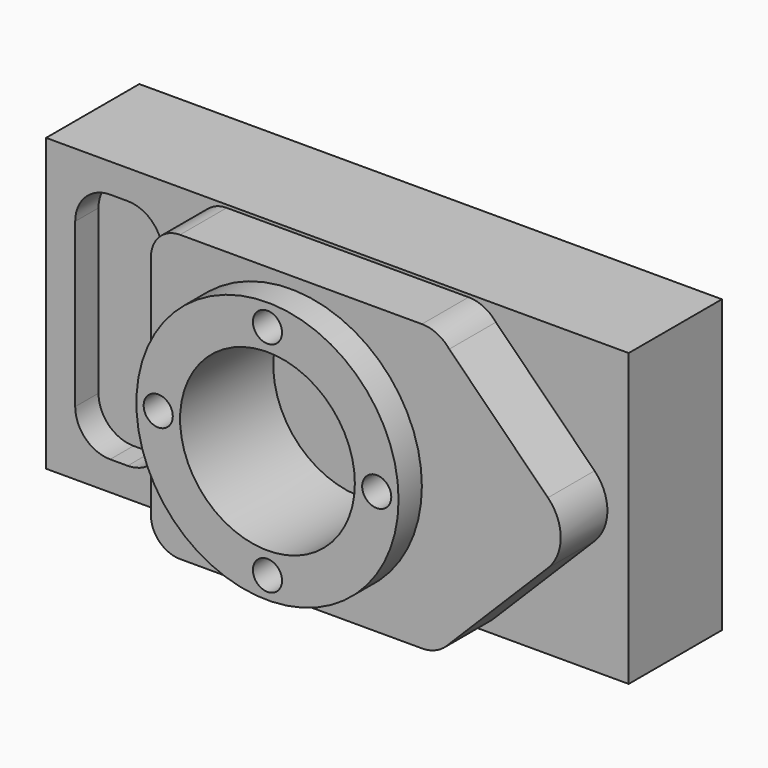
from build123d import *

# Parameters (mm, degrees)
F0_W     = 200
F0_H     = 100
F1_DEPTH = 40
F2_R     = 30
F3_DEPTH = 10
F4_R     = 30
F5_DEPTH = 20
F6_R     = 45
F6_R_2   = 30
F7_DEPTH = 10
F8_R     = 5
F9_DEPTH = 25


with BuildPart() as f1:
    # F0 (on Front) → F1 (new body)
    with BuildSketch(Plane.XZ):
        with Locations((-100, 50)):
            Rectangle(F0_W, F0_H)
    extrude(amount=F1_DEPTH)

    # F2 (on face) → F3 (cut)
    with BuildSketch(Plane.XZ.offset(40)):
        with BuildLine():
            Line((-172, 90), (-178, 90))
            ThreePointArc((-178, 90), (-186.4852813742, 86.4852813742), (-190, 78))
            Line((-190, 78), (-190, 22))
            ThreePointArc((-190, 22), (-186.4852813742, 13.5147186258), (-178, 10))
            Line((-178, 10), (-172, 10))
            ThreePointArc((-172, 10), (-163.5147186258, 13.5147186258), (-160, 22))
            Line((-160, 22), (-160, 78))
            ThreePointArc((-160, 78), (-163.5147186258, 86.4852813742), (-172, 90))
        make_face()
        with Locations((-100, 50)):
            Circle(F2_R)
    extrude(amount=-F3_DEPTH, mode=Mode.SUBTRACT)

    # F4 (on face) → F5 (join)
    with BuildSketch(Plane.XZ.offset(40)):
        with BuildLine():
            ThreePointArc((-138, 99), (-145.0710678119, 96.0710678119), (-148, 89))
            Line((-148, 89), (-148, 11))
            ThreePointArc((-148, 11), (-145.0710678119, 3.9289321881), (-138, 1))
            Line((-138, 1), (-54.98, 1))
            ThreePointArc((-54.98, 1), (-50.3814469261, 1.9160787793), (-46.485, 4.5244483955))
            Line((-46.485, 4.5244483955), (-11.6992693535, 39.39))
            ThreePointArc((-11.6992693535, 39.39), (-7.3180325381, 50.004327625), (-11.7274004602, 60.607))
            Line((-11.7274004602, 60.607), (-45.6005130737, 94.485))
            ThreePointArc((-45.6005130737, 94.485), (-49.7751945281, 97.8124927746), (-54.98, 99))
            Line((-54.98, 99), (-138, 99))
        make_face()
        with Locations((-100, 50)):
            Circle(F4_R, mode=Mode.SUBTRACT)
    extrude(amount=F5_DEPTH)

    # F6 (on face) → F7 (join)
    with BuildSketch(Plane.XZ.offset(60)):
        with Locations((-100, 50)):
            Circle(F6_R)
        with Locations((-100, 50)):
            Circle(F6_R_2, mode=Mode.SUBTRACT)
    extrude(amount=F7_DEPTH)

    # F8 (on face) → F9 (cut)
    with BuildSketch(Plane.XZ.offset(70)):
        with Locations((-100, 87.5)):
            Circle(F8_R)
        with Locations((-137.5, 50)):
            Circle(F8_R)
        with Locations((-100, 12.5)):
            Circle(F8_R)
        with Locations((-62.5, 50)):
            Circle(F8_R)
    extrude(amount=-F9_DEPTH, mode=Mode.SUBTRACT)


solid = f1.part
